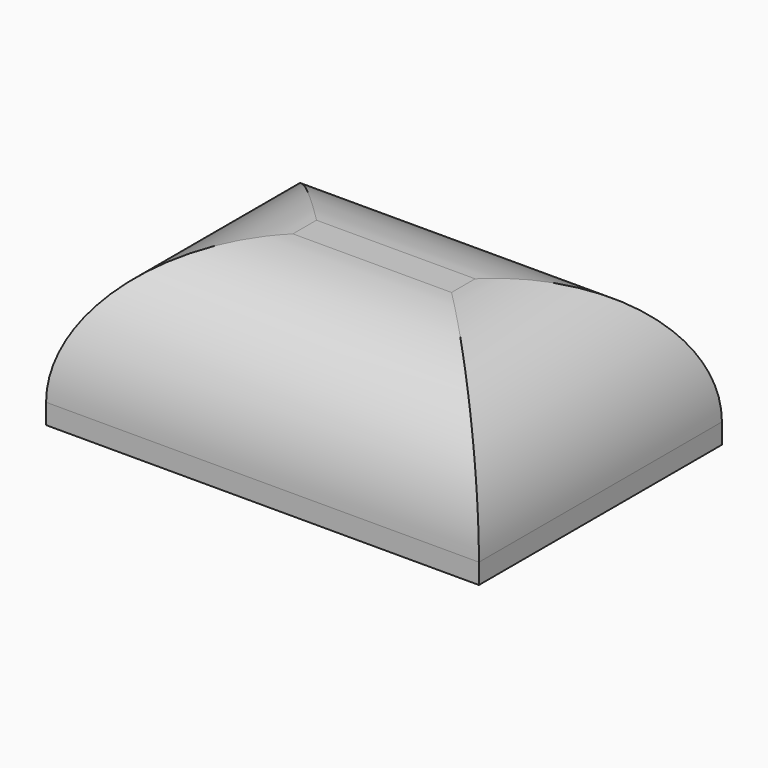
from build123d import *

# Parameters (mm, degrees)
F0_W     = 96.2325334549
F0_H     = 67.5312206149
F1_DEPTH = 34.95684
F2_R     = 30.48


# Not quite as in the source:
# - a feature names something its author has since deleted; it is built from what else it names


with BuildPart() as f1:
    # F0 (on Top) → F1 (new body)
    with BuildSketch(Plane.XY):
        with Locations((-48.1162667274, -33.7656103075)):
            Rectangle(F0_W, F0_H)
    extrude(amount=F1_DEPTH)

    # F2
    f2_edges = [f1.edges().sort_by_distance(p)[0] for p in [
        (0, -33.76561, 34.95684),
        (-48.116267, 0, 34.95684),
        (-96.232533, -33.76561, 34.95684),
        (-48.116267, -67.531221, 34.95684),
    ]]
    fillet(f2_edges, radius=F2_R)


solid = f1.part
